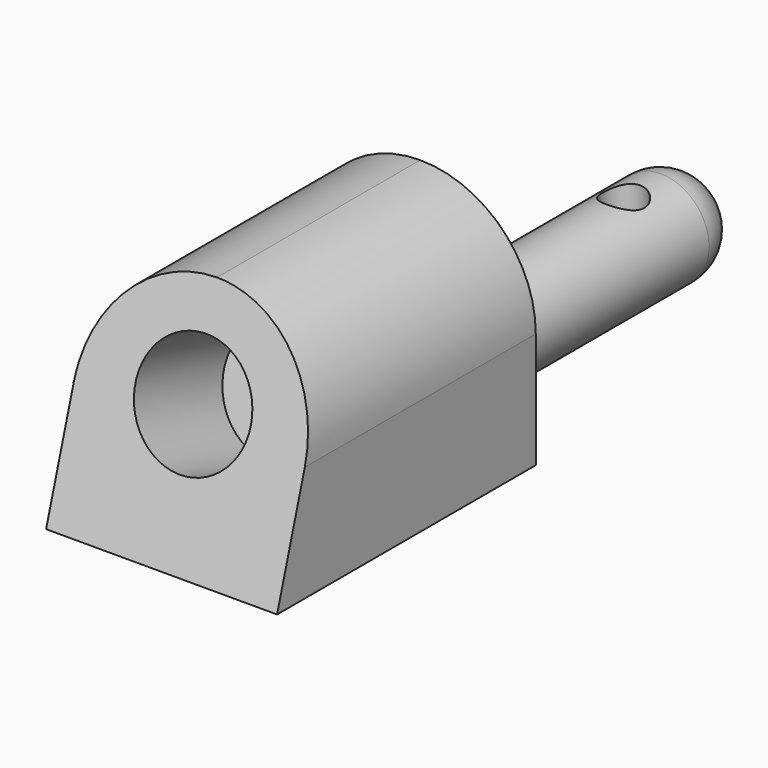
from build123d import *

# Parameters (mm, degrees)
F0_W      = 10
F0_H      = 14
F1_DEPTH  = 10
F2_R      = 2.1
F3_DEPTH  = 15
F4_R      = 0.9
F5_DEPTH  = 5
F6_R      = 2
F8_DEPTH  = 10
F9_R      = 2.5
F10_DEPTH = 5
F11_R     = 4.99999


# Not quite as in the source:
# - a fillet or chamfer is up to 0.001 mm smaller than in the source, because OpenCascade refuses the exact size


with BuildPart() as f1:
    # F0 (on Top) → F1 (new body)
    with BuildSketch(Plane.XY):
        Rectangle(F0_W, F0_H)
    extrude(amount=F1_DEPTH)

    # F2 (on face) → F3 (join)
    with BuildSketch(Plane(origin=(0, 7, 0), x_dir=(-1, 0, 0), z_dir=(0, 1, 0))):
        with Locations((0, 2.1)):
            Circle(F2_R)
    extrude(amount=F3_DEPTH)

    # F4 (on Top) → F5 (cut)
    with BuildSketch(Plane.XY):
        with Locations((0, 18)):
            Circle(F4_R)
    extrude(amount=F5_DEPTH, mode=Mode.SUBTRACT)

    # F6
    f6_edges = [f1.edges().sort_by_distance(p)[0] for p in [
        (2.1, 22, 2.1),
    ]]
    fillet(f6_edges, radius=F6_R)

    # F7 (on face) → F8 (cut)
    with BuildSketch(Plane(origin=(-5, 0, 0), x_dir=(0, -1, 0), z_dir=(-1, 0, 0))):
        Polygon((4, 10), (7, 0), (7, 10), align=None)
    extrude(amount=-F8_DEPTH, mode=Mode.SUBTRACT)

    # F9 (on face) → F10 (cut)
    with BuildSketch(Plane(origin=(0, -6.4220183486, 1.9266055046), x_dir=(1, 0, 0), z_dir=(0, -0.9578262852, 0.2873478856))):
        with Locations((0, 3.9318241179)):
            Circle(F9_R)
    extrude(amount=-F10_DEPTH, mode=Mode.SUBTRACT)

    # F11 (radius 5 in the source; OpenCascade refuses exactly that, so slightly less here)
    f11_edges = [f1.edges().sort_by_distance(p)[0] for p in [
        (-5, 1.5, 10),
        (5, 1.5, 10),
    ]]
    fillet(f11_edges, radius=F11_R)


solid = f1.part
